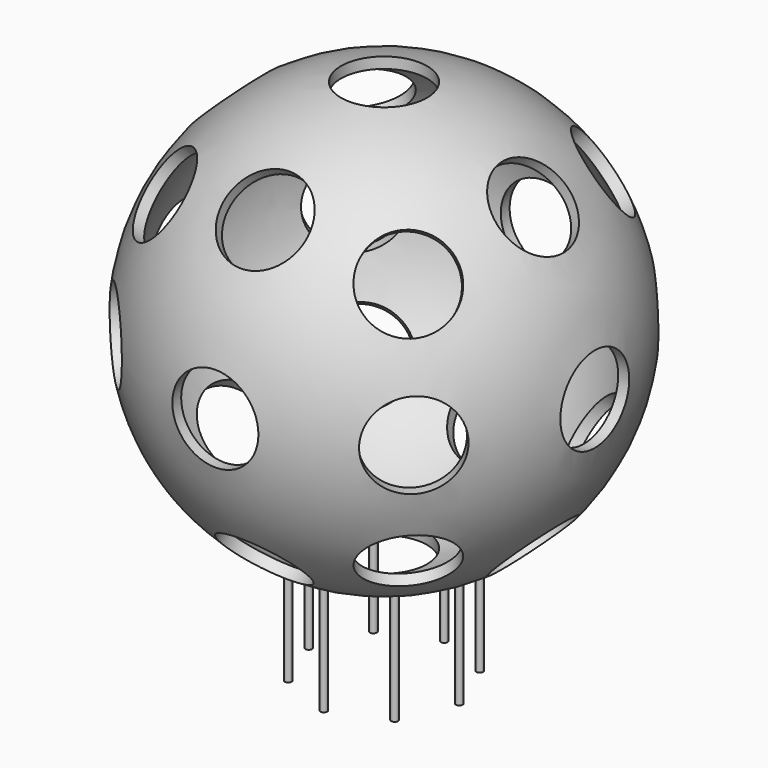
from build123d import *

# Parameters (mm, degrees)
F22_R            = 5.08
F23_DEPTH        = 38.1
F25_R            = 5.08
F26_DEPTH        = 38.1
F26_COPIES_COUNT = 6
F26_COPIES_ANGLE = 225
F28_R            = 5.08
F29_DEPTH        = 38.1
F54_R            = 5.08
F55_DEPTH        = 63.5
F55_COPIES_COUNT = 4
F73_R            = 5.08
F74_DEPTH        = 25.401
F76_R            = 0.4064
F77_DEPTH        = 13.97
F77_COPIES_COUNT = 8


# Not quite as in the source:
# - a feature of the source that left no trace in its solid (it failed there, or was rolled back) is left out
# - a pattern or mirror of a feature is missing from the dataset's text; its kind, count and spacing are read off the source's solid


with BuildPart() as f2:
    # F1 (on Top) → F2 (revolve)
    with BuildSketch(Plane.XY):
        with BuildLine():
            Line((0, -25.4), (0, 25.4))
            ThreePointArc((0, 25.4), (-25.4, 0), (0, -25.4))
        make_face()
    revolve(axis=Axis((0, 0, 0), (0, -1, 0)))

    # F22 (on plane+point) → F23 (cut, symmetric)
    with BuildSketch(Plane.XY.offset(25.4)):
        Circle(F22_R)
    f23 = extrude(amount=F23_DEPTH, both=True, mode=Mode.SUBTRACT)

    # F23_copies: F23 across plane
    add(f23.mirror(Plane(origin=(0, 0, 0), x_dir=(-0.8164965809, 0, -0.5773502692), z_dir=(0.5, 0.5, -0.7071067812))), mode=Mode.SUBTRACT)

    # F25 (on plane+point) → F26 (cut, symmetric)
    with BuildSketch(Plane.YZ.offset(25.4)):
        Circle(F25_R)
    f26 = extrude(amount=F26_DEPTH, both=True, mode=Mode.SUBTRACT)

    # F26_copies: F26 ×6 about axis
    f26_copies_axis = Axis((0, 0, 0), (0, 0, -1))
    for i in range(1, F26_COPIES_COUNT):
        add(f26.rotate(f26_copies_axis, i * F26_COPIES_ANGLE / (F26_COPIES_COUNT - 1)), mode=Mode.SUBTRACT)

    # F28 (on plane+point) → F29 (cut, symmetric)
    with BuildSketch(Plane.XZ.offset(-25.4)):
        Circle(F28_R)
    extrude(amount=F29_DEPTH, both=True, mode=Mode.SUBTRACT)

    # F42 (on Top) → F43 (revolve, cut)
    with BuildSketch(Plane.XY):
        with BuildLine():
            Line((0, -24.13), (0, 24.13))
            ThreePointArc((0, 24.13), (-24.13, 0), (0, -24.13))
        make_face()
    revolve(axis=Axis((0, 12.7, 0), (0, 1, 0)), mode=Mode.SUBTRACT)

    # F54 (on face) → F55 (cut, symmetric)
    with BuildSketch(Plane(origin=(7.3323484187, -7.3323484187, 7.3323484187), x_dir=(-0.8164965809, -0.4082482905, 0.4082482905), z_dir=(-0.5773502692, 0.5773502692, -0.5773502692))):
        Circle(F54_R)
    f55 = extrude(amount=F55_DEPTH, both=True, mode=Mode.SUBTRACT)

    # F55_copies: F55 ×4 about axis
    f55_copies_axis = Axis((0, 0, 0), (0, 0, 1))
    for i in range(1, F55_COPIES_COUNT):
        add(f55.rotate(f55_copies_axis, i * 360 / F55_COPIES_COUNT), mode=Mode.SUBTRACT)

    # F55_copies1: F55 across plane
    add(f55.mirror(Plane(origin=(0, 0, 0), x_dir=(0, -0.9120955865, -0.4099776106), z_dir=(0.0917517095, 0.4082482905, -0.9082482905))), mode=Mode.SUBTRACT)

    # F55_copies2: F55 across plane
    add(f55.mirror(Plane(origin=(0, 0, 0), x_dir=(0.9756630355, -0.2192752634, 0), z_dir=(0.2141864953, 0.9530206139, 0.2141864953))), mode=Mode.SUBTRACT)

    # F55_copies3: F55 across plane
    add(f55.mirror(Plane(origin=(0, 0, 0), x_dir=(-0.9117817457, 0, 0.4106751127), z_dir=(-0.4088667442, -0.09374123, -0.9077668022))), mode=Mode.SUBTRACT)

    # F55_copies4: F55 across plane
    add(f55.mirror(Plane(origin=(0, 0, 0), x_dir=(-0.2234726459, 0, -0.9747102013), z_dir=(-0.9530060831, -0.2098539363, 0.218496524))), mode=Mode.SUBTRACT)

    # F73 (on Top) → F74 (cut, through all)
    with BuildSketch(Plane.XY):
        Circle(F73_R)
    extrude(amount=-F74_DEPTH, mode=Mode.SUBTRACT)

    # F76 (on offset) → F77 (join)
    with BuildSketch(Plane.XY.offset(-22.86)):
        with Locations((0, -8.89)):
            Circle(F76_R)
    f77 = extrude(amount=-F77_DEPTH)

    # F77_copies: F77 ×8 about axis
    f77_copies_axis = Axis((0, 0, 0), (0, 0, 1))
    for i in range(1, F77_COPIES_COUNT):
        add(f77.rotate(f77_copies_axis, i * 360 / F77_COPIES_COUNT))


solid = f2.part
